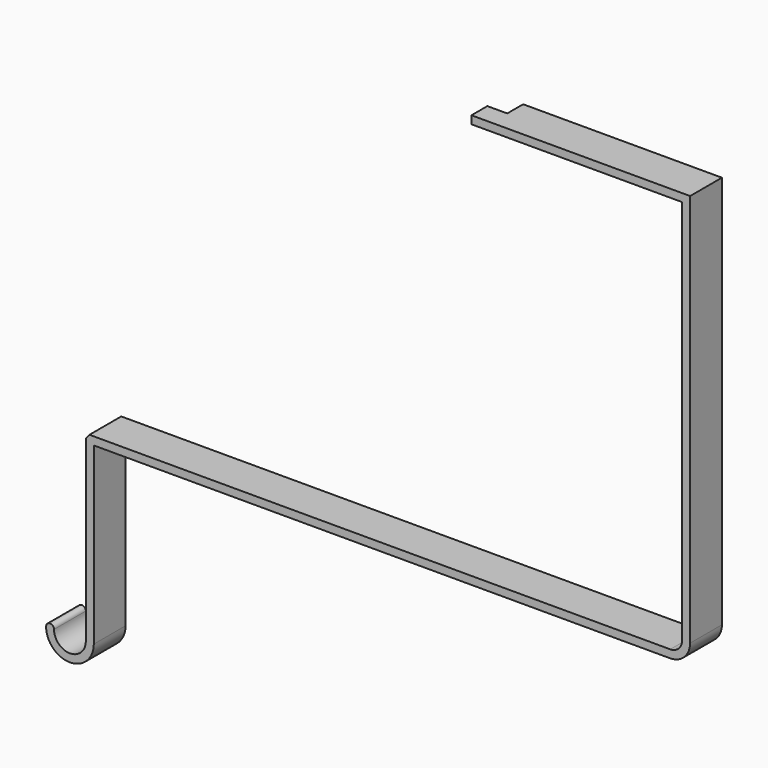
from build123d import *

# Parameters (mm, degrees)
F1_DEPTH = 5
F0_W     = 5
F0_H     = 2
F2_DEPTH = 5


# Not quite as in the source:
# - ends of sketch curves that miss each other by under 0.0002 mm in the source are joined


with BuildPart() as f1:
    # F0 (on Front) → F1 (new body, symmetric)
    with BuildSketch(Plane.XZ):
        with BuildLine():
            Line((103.7702985108, 110.5688567758), (53.7702985108, 110.5688567758))
            Line((53.7702985108, 110.5688567758), (53.7702985108, 108.5688567758))
            Line((53.7702985108, 108.5688567758), (101.7702985108, 108.5688567758))
            Line((101.7702985108, 108.5688567758), (101.7702985108, 11.5688567758))
            ThreePointArc((101.7702985108, 11.5688567758), (100.8916188543, 9.4475364322), (98.7702985108, 8.5688567758))
            Line((98.7702985108, 8.5688567758), (-47.322679311, 8.5688567758))
            Line((-47.322679311, 8.5688567758), (-48.2297014892, 7.4968221597))
            Line((-48.2297014892, 7.4968221597), (-48.2297014892, -37.4311432242))
            ThreePointArc((-48.2297014892, -37.4311432242), (-52.2297014892, -41.4311438799), (-56.2297021449, -37.4311432242))
            ThreePointArc((-56.2297021449, -37.4311432242), (-57.229701817, -36.4311435521), (-58.2297014892, -37.4311432242))
            ThreePointArc((-58.2297014892, -37.4311432242), (-52.2297014892, -43.4311432242), (-46.2297014892, -37.4311432242))
            Line((-46.2297014892, -37.4311432242), (-46.2297014892, 6.5688567758))
            Line((-46.2297014892, 6.5688567758), (98.7702985108, 6.5688567758))
            ThreePointArc((98.7702985108, 6.5688567758), (102.3058324167, 8.0333228698), (103.7702985108, 11.5688567758))
            Line((103.7702985108, 11.5688567758), (103.7702985108, 110.5688567758))
        make_face()
    extrude(amount=F1_DEPTH, both=True)

    # F0 (on Front) → F2 (join)
    with BuildSketch(Plane.XZ):
        with Locations((51.2702985108, 109.5688567758)):
            Rectangle(F0_W, F0_H)
    extrude(amount=F2_DEPTH)


solid = f1.part
